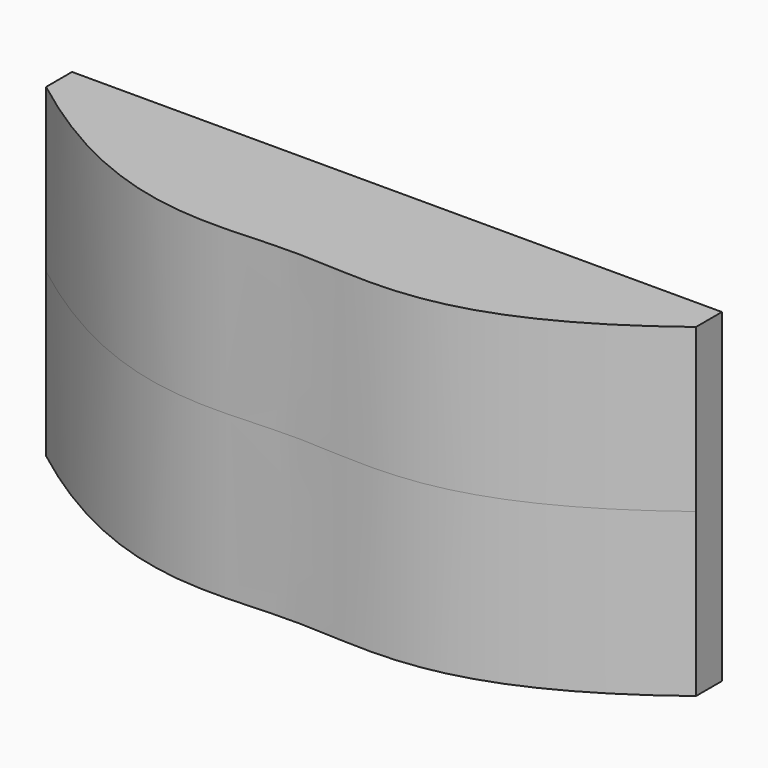
from build123d import *

# Parameters (mm, degrees)
F1_DEPTH         = 50
F2_T             = -2.5
F4_COPIES2_COUNT = 2


# Not quite as in the source:
# - a pattern or mirror of a feature is missing from the dataset's text; its kind, count and spacing are read off the source's solid


with BuildPart() as f1:
    # F0 (on Top) → F1 (new body, symmetric)
    with BuildSketch(Plane.XY):
        with BuildLine():
            Line((100, 0), (100, 9.9865811612))
            Line((100, 9.9865811612), (-100, 9.9865811612))
            Line((-100, 9.9865811612), (-100, 0))
            add(Edge.make_bspline(
                [(-100, 0), (-50, -38.3344968985), (0, -21.6655031015), (50, -38.3344968985), (100, 0)],
                knots=[0, 0, 0, 0, 0.5, 1, 1, 1, 1], degree=3))
        make_face()
    extrude(amount=F1_DEPTH, both=True)

    # F2
    f2_openings = [f1.faces().sort_by_distance(p)[0] for p in [
        (0, 9.986581, 0),
    ]]
    offset(amount=F2_T, openings=f2_openings, kind=Kind.INTERSECTION)


with BuildPart() as f4:
    # F3 (on face) → F4 (new body, up to the next surface of F1)
    with BuildSketch(Plane(origin=(0, 9.9865811612, 0), x_dir=(-1, 0, 0), z_dir=(0, 1, 0))):
        with BuildLine():
            ThreePointArc((97.5, 41.5138781887), (94.8743686708, 44.8743686708), (91.5138781887, 47.5))
            Line((91.5138781887, 47.5), (82.5, 47.5))
            Line((82.5, 47.5), (73.4861218113, 47.5))
            ThreePointArc((73.4861218113, 47.5), (70.1256313292, 20.1256313292), (97.5, 23.4861218113))
            Line((97.5, 23.4861218113), (97.5, 41.5138781887))
        make_face()
        with BuildLine():
            ThreePointArc((90, 32.5), (77.1966991411, 27.1966991411), (82.5, 40))
            ThreePointArc((82.5, 40), (87.8033008589, 37.8033008589), (90, 32.5))
        make_face(mode=Mode.SUBTRACT)
    extrude(until=Until.NEXT, target=f1.part, dir=(0, -1, 0))


with BuildPart() as f4_copies_1:
    # F4_copies: instance of F4
    add(f4.part.mirror(Plane(origin=(0, 0, -5e-06), x_dir=(-1, 0, 0), z_dir=(0, 0, -1))))


with BuildPart() as f4_copies1_1:
    # F4_copies1: instance of F4
    add(f4.part.mirror(Plane(origin=(2e-06, 0, 0), x_dir=(0, 0, 1), z_dir=(1, 0, 0))))


with BuildPart() as f4_copies2_1:
    # F4_copies2: instance of F4
    add(f4.part.rotate(Axis((0, 0, 0), (0, 1, 0)), 1 * 360 / F4_COPIES2_COUNT))


solid = Compound([f1.part, f4.part, f4_copies_1.part, f4_copies1_1.part, f4_copies2_1.part])
